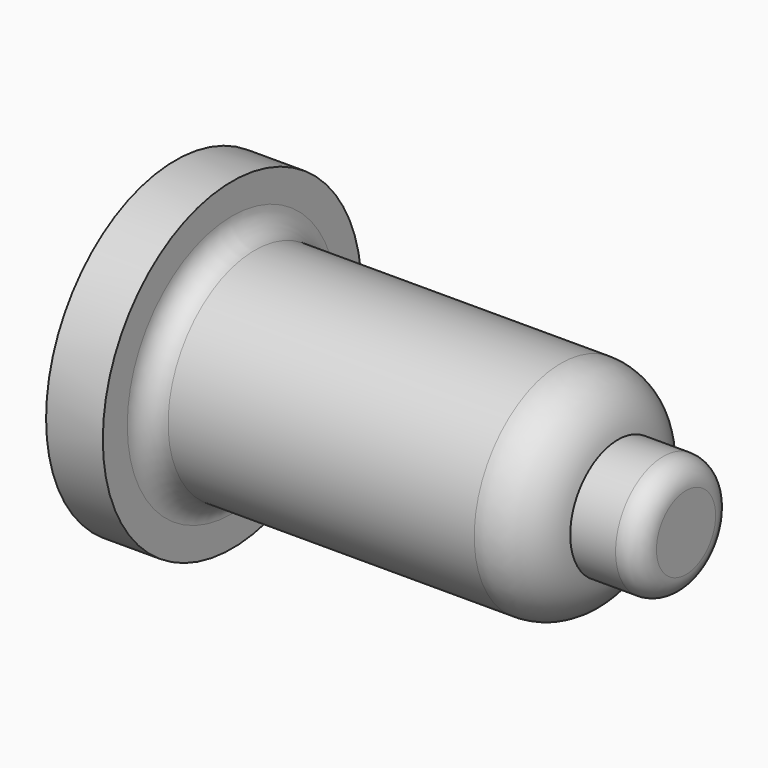
from build123d import *

# Parameters (mm, degrees)
F0_R      = 5.258166692
F12_DEPTH = 45
F1_R      = 9.5550685652
F2_DEPTH  = 39
F13_R     = 14.2505021401
F3_DEPTH  = 5
F4_R      = 2
F6_R      = 2
F10_W     = 1.8654689193
F10_H     = 2.0018368959
F11_DEPTH = 45


# Not quite as in the source:
# - a fillet or chamfer that OpenCascade refuses, or shapes differently, is made with other operations: its cross-section is extruded or revolved along the edge and cut away or added
# - the program builds the solid bodies; features that only make, move or delete a surface that nothing else refers to are left out


with BuildPart() as f12:
    # F0 (on Right) → F12 (new body)
    with BuildSketch(Plane.YZ):
        Circle(F0_R)
    extrude(amount=F12_DEPTH)

    # F1 (on Right) → F2 (join)
    with BuildSketch(Plane.YZ):
        Circle(F1_R)
    extrude(amount=F2_DEPTH)

    # F13 (on Right) → F3 (join)
    with BuildSketch(Plane.YZ):
        Circle(F13_R)
    extrude(amount=F3_DEPTH)

    # F4
    f4_edges = [f12.edges().sort_by_distance(p)[0] for p in [
        (45, -5.258167, 0),
    ]]
    fillet(f4_edges, radius=F4_R)

    # F5: fillet of radius 5.08 on 1 edges, made by hand

    # F5_s1 → F5_t2 (revolve, cut)
    with BuildSketch(Plane.XY):
        with BuildLine():
            ThreePointArc((39, 5.258166692), (37.2843755862, 8.3341188683), (33.9807214339, 9.5550685652))
            Line((33.9807214339, 9.5550685652), (39, 9.5550685652))
            Line((39, 9.5550685652), (39, 5.258166692))
        make_face()
    revolve(axis=Axis((39, 0, 0), (1, 0, 0)), mode=Mode.SUBTRACT)

    # F6
    f6_edges = [f12.edges().sort_by_distance(p)[0] for p in [
        (5, -9.555069, 0),
    ]]
    fillet(f6_edges, radius=F6_R)

    # F10 (on Right) → F11 (join)
    with BuildSketch(Plane.YZ):
        Rectangle(F10_W, F10_H)
    extrude(amount=F11_DEPTH)


solid = f12.part
